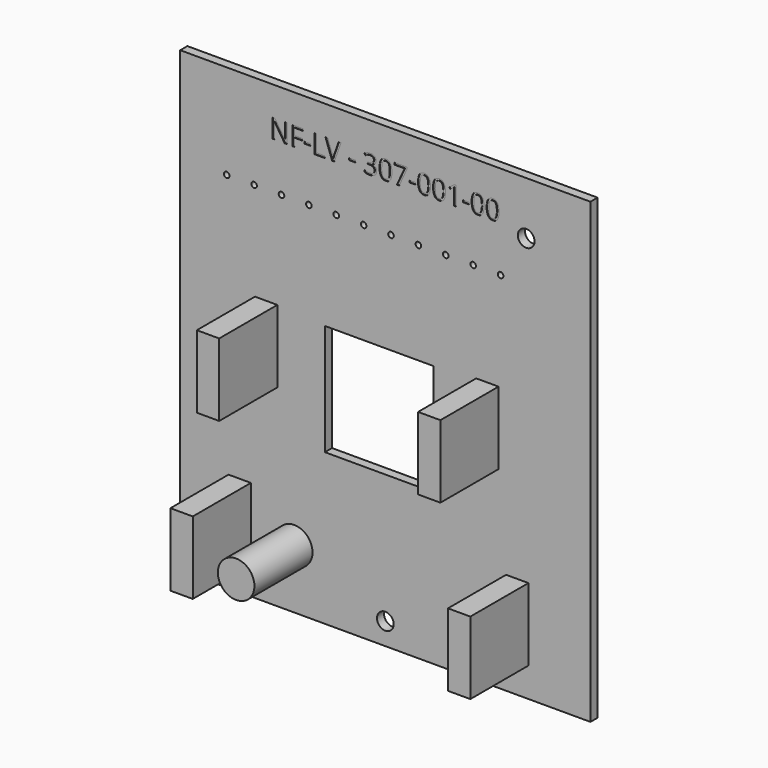
from build123d import *

# Parameters (mm, degrees)
F0_W         = 73.4
F0_H         = 81.9407834101
F0_W_2       = 4
F0_H_2       = 13
F0_R         = 3.2698799256
F0_W_3       = 19.4679377601
F0_H_3       = 19.886600785
F0_R_2       = 1.5
F0_R_3       = 0.5
F1_DEPTH     = 1.6
F2_TEXT_SIZE = 4.7043017629
F3_DEPTH     = 0.1
F4_DEPTH     = 13


# Not quite as in the source:
# - Text() gives the source's letters only with a copy of the font that has no kerning and outlines rounded to 1/6400 em; it was checked with that copy


with BuildPart() as f1:
    # F0 (on Front) → F1 (new body)
    with BuildSketch(Plane.XZ):
        Rectangle(F0_W, F0_H)
        with Locations((-26.0564852506, -29.5752882957)):
            Rectangle(F0_W_2, F0_H_2, mode=Mode.SUBTRACT)
        with Locations((-16.2955727428, -30.4479897022)):
            Circle(F0_R, mode=Mode.SUBTRACT)
        with Locations((-1.0804939084, -3.9884527214)):
            Rectangle(F0_W_3, F0_H_3, mode=Mode.SUBTRACT)
        with Locations((0, -37.0434857905)):
            Circle(F0_R_2, mode=Mode.SUBTRACT)
        with Locations((23.6070174724, -29.2018782347)):
            Rectangle(F0_W_2, F0_H_2, mode=Mode.SUBTRACT)
        with Locations((-21.3266275823, 0)):
            Rectangle(F0_W_2, F0_H_2, mode=Mode.SUBTRACT)
        with Locations((-28.3819679171, 24.0354221314)):
            Circle(F0_R_3, mode=Mode.SUBTRACT)
        with Locations((-23.4819937642, 24.0513375523)):
            Circle(F0_R_3, mode=Mode.SUBTRACT)
        with Locations((-18.5820196112, 24.0672529731)):
            Circle(F0_R_3, mode=Mode.SUBTRACT)
        with Locations((-13.6820454583, 24.083168394)):
            Circle(F0_R_3, mode=Mode.SUBTRACT)
        with Locations((-8.7820713054, 24.0990838149)):
            Circle(F0_R_3, mode=Mode.SUBTRACT)
        with Locations((-3.8820971524, 24.1149992357)):
            Circle(F0_R_3, mode=Mode.SUBTRACT)
        with Locations((18.2548090816, 0)):
            Rectangle(F0_W_2, F0_H_2, mode=Mode.SUBTRACT)
        with Locations((1.0178770005, 24.1309146566)):
            Circle(F0_R_3, mode=Mode.SUBTRACT)
        with Locations((5.9178511534, 24.1468300774)):
            Circle(F0_R_3, mode=Mode.SUBTRACT)
        with Locations((10.8178253064, 24.1627454983)):
            Circle(F0_R_3, mode=Mode.SUBTRACT)
        with Locations((15.7177994593, 24.1786609191)):
            Circle(F0_R_3, mode=Mode.SUBTRACT)
        with Locations((20.6177736122, 24.19457634)):
            Circle(F0_R_3, mode=Mode.SUBTRACT)
        with Locations((25.2, 31.4703917051)):
            Circle(F0_R_2, mode=Mode.SUBTRACT)
        with Locations((-21.3266275823, 0)):
            Rectangle(F0_W_2, F0_H_2)
        with Locations((18.2548090816, 0)):
            Rectangle(F0_W_2, F0_H_2)
        with Locations((23.6070174724, -29.2018782347)):
            Rectangle(F0_W_2, F0_H_2)
        with Locations((-16.2955727428, -30.4479897022)):
            Circle(F0_R)
        with Locations((-26.0564852506, -29.5752882957)):
            Rectangle(F0_W_2, F0_H_2)
    extrude(amount=-F1_DEPTH)

    # F2 (on face) → F3 (cut)
    with BuildSketch(Plane.XZ):
        with Locations((-20.651149692, 32.3891155422)):
            Text('NF-LV - 307-001-00', F2_TEXT_SIZE, font='Open Sans', text_align=(TextAlign.LEFT, TextAlign.BOTTOM))
    extrude(amount=-F3_DEPTH, mode=Mode.SUBTRACT)

    # F0 (on Front) → F4 (join)
    with BuildSketch(Plane.XZ):
        with Locations((-21.3266275823, 0)):
            Rectangle(F0_W_2, F0_H_2)
        with Locations((18.2548090816, 0)):
            Rectangle(F0_W_2, F0_H_2)
        with Locations((-16.2955727428, -30.4479897022)):
            Circle(F0_R)
        with Locations((-26.0564852506, -29.5752882957)):
            Rectangle(F0_W_2, F0_H_2)
        with Locations((23.6070174724, -29.2018782347)):
            Rectangle(F0_W_2, F0_H_2)
    extrude(amount=F4_DEPTH)


solid = f1.part
